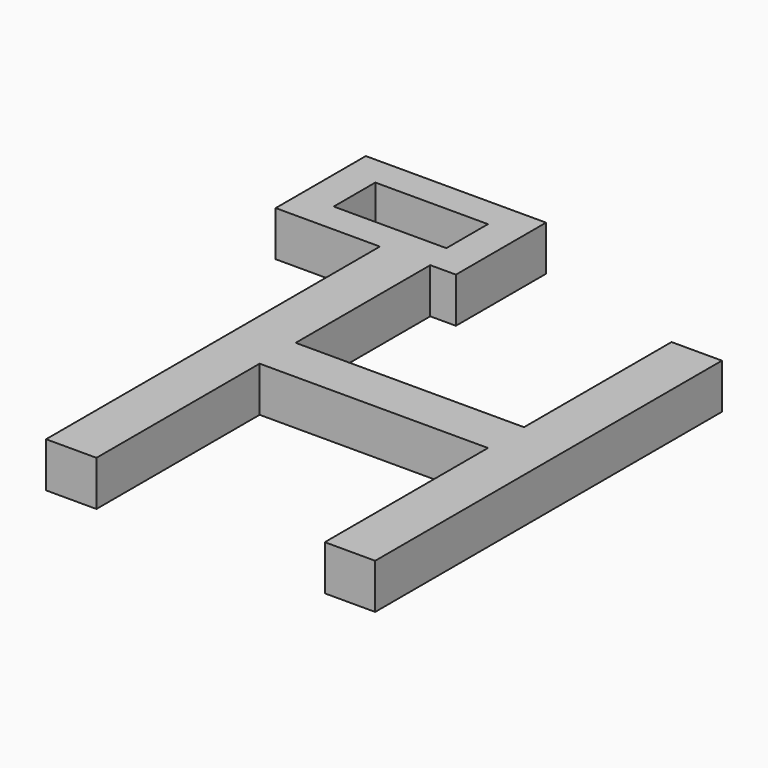
from build123d import *

# Parameters (mm, degrees)
F0_W     = 2.236037234
F0_H     = 0.718915021
F1_DEPTH = 2


with BuildPart() as f1:
    # F0 (on Top) → F1 (new body)
    with BuildSketch(Plane.XY):
        Polygon((2.0192633942, 0.4625715956), (2.0192633942, -0.8831437444), (2.6445035461, -0.8831437444), (2.6445035461, -0.1642287234), (4.8805407801, -0.1642287234), (4.8805407801, -0.8831437444), (6.0192633942, -0.8831437444), (6.0192633942, 4.1168562556), (2.0192633942, 4.1168562556), (2.0192633942, 2.7711409156), (4.5192633942, 2.7711409156), (4.5192633942, 0.4625715956), align=None)
        Polygon((-1.9807366058, -0.8831437444), (2.0192633942, -0.8831437444), (2.0192633942, 0.4625715956), (-0.4807366058, 0.4625715956), (-0.4807366058, 2.7711409156), (2.0192633942, 2.7711409156), (2.0192633942, 4.1168562556), (-1.9807366058, 4.1168562556), align=None)
        with Locations((3.7625221631, -0.5236862339)):
            Rectangle(F0_W, F0_H)
        Polygon((4.8805407801, -0.8831437444), (2.6445035461, -0.8831437444), (2.6445035461, -19.4042553191), (4.8805407801, -19.4042553191), (4.8805407801, -10.3506205674), (15.0164007092, -10.3506205674), (15.0164007092, -19.4042553191), (17.2524379433, -19.4042553191), (17.2524379433, -0.1642287234), (15.0164007092, -0.1642287234), (15.0164007092, -8.3503989362), (4.8805407801, -8.3503989362), align=None)
    extrude(amount=F1_DEPTH)


solid = f1.part
